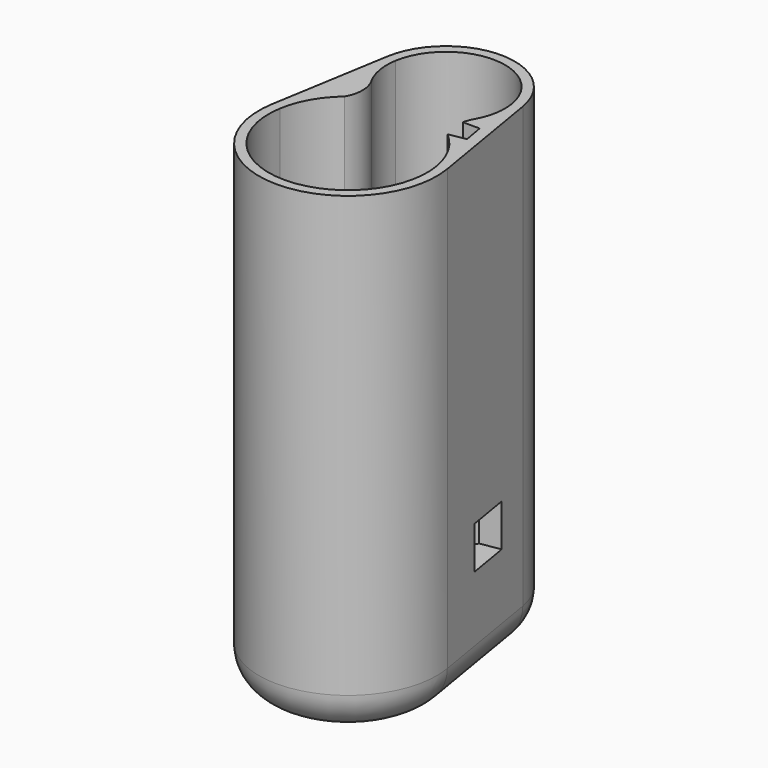
from build123d import *

# Parameters (mm, degrees)
F1_DEPTH    = 71.5
F0_R        = 0.8
F2_DEPTH    = 3
F3_T1_DEPTH = 18.8384580048
F3_T3_DEPTH = 18.8384580048
F3_T6_ANGLE = 198.9853445977
F3_T8_ANGLE = 161.0146554023
F6_W        = 6.8
F6_H        = 6.6
F7_DEPTH    = 10
F9_DEPTH    = 57.4


# Not quite as in the source:
# - a fillet or chamfer that OpenCascade refuses, or shapes differently, is made with other operations: its cross-section is extruded or revolved along the edge and cut away or added


with BuildPart() as f1:
    # F0 (on Top) → F1 (new body)
    with BuildSketch(Plane.XY):
        with BuildLine():
            ThreePointArc((10.5534817095, 15.4336250836), (0, 24.3689653978), (-10.5534817095, 15.4336250836))
            Line((-10.5534817095, 15.4336250836), (-13.6603478203, -3.1468722986))
            ThreePointArc((-13.6603478203, -3.1468722986), (0, -19.2810346022), (13.6603478203, -3.1468722986))
            Line((13.6603478203, -3.1468722986), (10.5534817095, 15.4336250836))
        make_face()
        with BuildLine():
            ThreePointArc((-12.1808877675, -3.3942544975), (-10.7458713669, 0.6557337165), (-8.0101498113, 3.9689653978))
            ThreePointArc((-8.0101498113, 3.9689653978), (-7.3298242511, 6.556361809), (-8.0101498113, 9.1437582202))
            ThreePointArc((-8.0101498113, 9.1437582202), (-9.0606365073, 12.0737017575), (-9.0740216568, 15.1862428847))
            ThreePointArc((-9.0740216568, 15.1862428847), (0, 22.8689653978), (9.0740216568, 15.1862428847))
            ThreePointArc((9.0740216568, 15.1862428847), (9.0606535532, 12.0737985759), (8.0102465186, 9.1439294077))
            ThreePointArc((8.0102465186, 9.1439294077), (8.0101981654, 9.1438438137), (8.0101498113, 9.1437582202))
            ThreePointArc((8.0101498113, 9.1437582202), (7.3298242511, 6.556361809), (8.0101498113, 3.9689653978))
            ThreePointArc((8.0101498113, 3.9689653978), (10.7458713669, 0.6557337165), (12.1808877675, -3.3942544975))
            ThreePointArc((12.1808877675, -3.3942544975), (0, -17.7810346022), (-12.1808877675, -3.3942544975))
        make_face(mode=Mode.SUBTRACT)
    extrude(amount=F1_DEPTH)

    # F0 (on Top) → F2 (join)
    with BuildSketch(Plane.XY):
        with BuildLine():
            ThreePointArc((10.5534817095, 15.4336250836), (0, 24.3689653978), (-10.5534817095, 15.4336250836))
            Line((-10.5534817095, 15.4336250836), (-13.6603478203, -3.1468722986))
            ThreePointArc((-13.6603478203, -3.1468722986), (0, -19.2810346022), (13.6603478203, -3.1468722986))
            Line((13.6603478203, -3.1468722986), (10.5534817095, 15.4336250836))
        make_face()
        with BuildLine():
            ThreePointArc((-12.1808877675, -3.3942544975), (-10.7458713669, 0.6557337165), (-8.0101498113, 3.9689653978))
            ThreePointArc((-8.0101498113, 3.9689653978), (-7.3298242511, 6.556361809), (-8.0101498113, 9.1437582202))
            ThreePointArc((-8.0101498113, 9.1437582202), (-9.0606365073, 12.0737017575), (-9.0740216568, 15.1862428847))
            ThreePointArc((-9.0740216568, 15.1862428847), (0, 22.8689653978), (9.0740216568, 15.1862428847))
            ThreePointArc((9.0740216568, 15.1862428847), (9.0606535532, 12.0737985759), (8.0102465186, 9.1439294077))
            ThreePointArc((8.0102465186, 9.1439294077), (8.0101981654, 9.1438438137), (8.0101498113, 9.1437582202))
            ThreePointArc((8.0101498113, 9.1437582202), (7.3298242511, 6.556361809), (8.0101498113, 3.9689653978))
            ThreePointArc((8.0101498113, 3.9689653978), (10.7458713669, 0.6557337165), (12.1808877675, -3.3942544975))
            ThreePointArc((12.1808877675, -3.3942544975), (0, -17.7810346022), (-12.1808877675, -3.3942544975))
        make_face(mode=Mode.SUBTRACT)
        with BuildLine():
            ThreePointArc((-9.0740216568, 15.1862428847), (-9.0606365073, 12.0737017575), (-8.0101498113, 9.1437582202))
            ThreePointArc((-8.0101498113, 9.1437582202), (0, 4.4689653978), (8.0101498113, 9.1437582202))
            ThreePointArc((8.0101498113, 9.1437582202), (8.0101981654, 9.1438438137), (8.0102465186, 9.1439294077))
            ThreePointArc((8.0102465186, 9.1439294077), (9.0606535532, 12.0737985759), (9.0740216568, 15.1862428847))
            ThreePointArc((9.0740216568, 15.1862428847), (0, 22.8689653978), (-9.0740216568, 15.1862428847))
        make_face()
        with BuildLine():
            ThreePointArc((-8.0101498113, 9.1437582202), (-7.3298242511, 6.556361809), (-8.0101498113, 3.9689653978))
            Line((-8.0101498113, 3.9689653978), (8.0101498113, 3.9689653978))
            ThreePointArc((8.0101498113, 3.9689653978), (7.3298242511, 6.556361809), (8.0101498113, 9.1437582202))
            ThreePointArc((8.0101498113, 9.1437582202), (0, 4.4689653978), (-8.0101498113, 9.1437582202))
        make_face()
        with BuildLine():
            Line((8.0101498113, 3.9689653978), (-8.0101498113, 3.9689653978))
            ThreePointArc((-8.0101498113, 3.9689653978), (-10.7458713669, 0.6557337165), (-12.1808877675, -3.3942544975))
            ThreePointArc((-12.1808877675, -3.3942544975), (0, -17.7810346022), (12.1808877675, -3.3942544975))
            ThreePointArc((12.1808877675, -3.3942544975), (10.7458713669, 0.6557337165), (8.0101498113, 3.9689653978))
        make_face()
        with Locations((-9, -5.4310346022)):
            Circle(F0_R, mode=Mode.SUBTRACT)
        with Locations((9, -5.4310346022)):
            Circle(F0_R, mode=Mode.SUBTRACT)
    extrude(amount=-F2_DEPTH)

    # F3: fillet of radius 6 on 1 edges, made by hand

    # F3_s2 → F3_t1 (cut)
    with BuildSketch(Plane(origin=(2.22343693, 13.2971819786, 0), x_dir=(0, 0, 1), z_dir=(-0.164921466, -0.9863067018, 0))):
        with BuildLine():
            ThreePointArc((-3, 6.9543058117), (-1.2426406871, 11.1969464988), (3, 12.9543058117))
            Line((3, 12.9543058117), (-3, 12.9543058117))
            Line((-3, 12.9543058117), (-3, 6.9543058117))
        make_face()
    extrude(amount=F3_T1_DEPTH, mode=Mode.SUBTRACT)

    # F3_s4 → F3_t3 (cut)
    with BuildSketch(Plane(origin=(0.8834291807, -5.2833154036, 0), x_dir=(0, 0, 1), z_dir=(-0.164921466, 0.9863067018, 0))):
        with BuildLine():
            ThreePointArc((3, 12.9543058117), (-1.2426406871, 11.1969464988), (-3, 6.9543058117))
            Line((-3, 6.9543058117), (-3, 12.9543058117))
            Line((-3, 12.9543058117), (3, 12.9543058117))
        make_face()
    extrude(amount=F3_T3_DEPTH, mode=Mode.SUBTRACT)

    # F3_s5 → F3_t6 (revolve, cut)
    with BuildSketch(Plane(origin=(-0.8834291807, -5.2833154036, 0), x_dir=(0, 0, 1), z_dir=(0.164921466, 0.9863067018, 0))):
        with BuildLine():
            ThreePointArc((-3, -6.9543058117), (-1.2426406871, -11.1969464988), (3, -12.9543058117))
            Line((3, -12.9543058117), (-3, -12.9543058117))
            Line((-3, -12.9543058117), (-3, -6.9543058117))
        make_face()
    revolve(axis=Axis((0, -5.4310346022, -3), (0, 0, 1)), revolution_arc=F3_T6_ANGLE, mode=Mode.SUBTRACT)

    # F3_s7 → F3_t8 (revolve, cut)
    with BuildSketch(Plane(origin=(-2.22343693, 13.2971819786, 0), x_dir=(0, 0, 1), z_dir=(0.164921466, -0.9863067018, 0))):
        with BuildLine():
            ThreePointArc((-3, -6.9543058117), (-1.2426406871, -11.1969464988), (3, -12.9543058117))
            Line((3, -12.9543058117), (-3, -12.9543058117))
            Line((-3, -12.9543058117), (-3, -6.9543058117))
        make_face()
    revolve(axis=Axis((0, 13.6689653978, -3), (0, 0, 1)), revolution_arc=F3_T8_ANGLE, mode=Mode.SUBTRACT)

    # F6 (on face) → F7 (cut)
    with BuildSketch(Plane(origin=(12.7769186395, 2.1364431051, 0), x_dir=(-0.164921466, 0.9863067018, 0), z_dir=(0.9863067018, 0.164921466, 0))):
        with Locations((4.8267343795, 16.4621602923)):
            Rectangle(F6_W, F6_H)
    extrude(amount=-F7_DEPTH, mode=Mode.SUBTRACT)

    # F8 (on face) → F9 (cut)
    with BuildSketch(Plane.XY.offset(71.5)):
        with BuildLine():
            Line((10.0688748062, 7.6421294361), (7.4430989219, 7.6421294361))
            ThreePointArc((7.4430989219, 7.6421294361), (7.3876854798, 5.7782940298), (7.9859788071, 4.0122254677))
            Line((7.9859788071, 4.0122254677), (10.6296725571, 4.4812676497))
            Line((10.6296725571, 4.4812676497), (10.0688748062, 7.6421294361))
        make_face()
    extrude(amount=-F9_DEPTH, mode=Mode.SUBTRACT)


solid = f1.part
